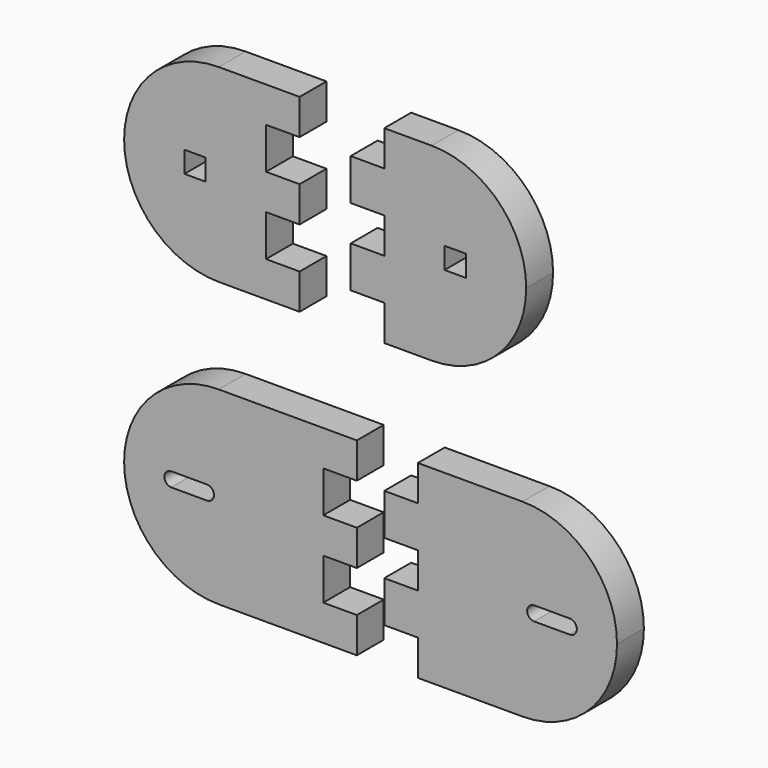
from build123d import *

# Parameters (mm, degrees)
F1_W     = 11.43
F1_H     = 11.43
F1_W_2   = 18.034
F1_H_2   = 19.05
F2_DEPTH = 18.034
F1_H_3   = 22.225


# Not quite as in the source:
# - a variable given as a bare number and used for a length is read in inches; the dataset says mm whatever the document's units were
# - a feature names something its author has since deleted; it is built from what else it names


with BuildPart() as f2:
    # F1 (on Front) → F2 (new body)
    with BuildSketch(Plane.XZ):
        with BuildLine():
            Line((-25.4, 0), (0, 0))
            Line((0, 0), (0, 19.05))
            Line((0, 19.05), (0, 41.275))
            Line((0, 41.275), (0, 60.325))
            Line((0, 60.325), (0, 82.55))
            Line((0, 82.55), (0, 101.6))
            Line((0, 101.6), (-25.4, 101.6))
            ThreePointArc((-25.4, 101.6), (-61.3210244843, 86.7210244843), (-76.2, 50.8))
            ThreePointArc((-76.2, 50.8), (-61.3210244843, 14.8789755157), (-25.4, 0))
        make_face()
        with Locations((-38.1, 50.8)):
            Rectangle(F1_W, F1_H, mode=Mode.SUBTRACT)
        with Locations((9.017, 92.075)):
            Rectangle(F1_W_2, F1_H_2)
        with Locations((9.017, 50.8)):
            Rectangle(F1_W_2, F1_H_2)
        with Locations((9.017, 9.525)):
            Rectangle(F1_W_2, F1_H_2)
    extrude(amount=F2_DEPTH)


with BuildPart() as f2b:
    # F1 (on Front) → F2, piece 2 (new body)
    with BuildSketch(Plane.XZ):
        with Locations((54.483, 30.1625)):
            Rectangle(F1_W_2, F1_H_3)
        with Locations((54.483, 71.4375)):
            Rectangle(F1_W_2, F1_H_3)
        with BuildLine():
            ThreePointArc((139.7, 50.8), (124.8210244843, 86.7210244843), (88.9, 101.6))
            Line((88.9, 101.6), (63.5, 101.6))
            Line((63.5, 101.6), (63.5, 82.55))
            Line((63.5, 82.55), (63.5, 60.325))
            Line((63.5, 60.325), (63.5, 41.275))
            Line((63.5, 41.275), (63.5, 19.05))
            Line((63.5, 19.05), (63.5, 0))
            Line((63.5, 0), (88.9, 0))
            ThreePointArc((88.9, 0), (124.8210244843, 14.8789755157), (139.7, 50.8))
        make_face()
        with Locations((101.6, 50.8)):
            Rectangle(F1_W, F1_H, mode=Mode.SUBTRACT)
    extrude(amount=F2_DEPTH)


with BuildPart() as f2c:
    # F1 (on Front) → F2, piece 3 (new body)
    with BuildSketch(Plane.XZ):
        with Locations((39.751, -101.6)):
            Rectangle(F1_W_2, F1_H_2)
        with BuildLine():
            Line((30.734, -50.8), (-25.4, -50.8))
            ThreePointArc((-25.4, -50.8), (-61.3210244843, -65.6789755157), (-76.2, -101.6))
            ThreePointArc((-76.2, -101.6), (-61.3210244843, -137.5210244843), (-25.4, -152.4))
            Line((-25.4, -152.4), (30.734, -152.4))
            Line((30.734, -152.4), (30.734, -133.35))
            Line((30.734, -133.35), (30.734, -111.125))
            Line((30.734, -111.125), (30.734, -92.075))
            Line((30.734, -92.075), (30.734, -69.85))
            Line((30.734, -69.85), (30.734, -50.8))
        make_face()
        with BuildLine():
            Line((-31.75, -105.41), (-50.8, -105.41))
            ThreePointArc((-50.8, -105.41), (-54.61, -101.6), (-50.8, -97.79))
            Line((-50.8, -97.79), (-31.75, -97.79))
            ThreePointArc((-31.75, -97.79), (-27.94, -101.6), (-31.75, -105.41))
        make_face(mode=Mode.SUBTRACT)
        with Locations((39.751, -142.875)):
            Rectangle(F1_W_2, F1_H_2)
        with Locations((39.751, -60.325)):
            Rectangle(F1_W_2, F1_H_2)
    extrude(amount=F2_DEPTH)


with BuildPart() as f2d:
    # F1 (on Front) → F2, piece 4 (new body)
    with BuildSketch(Plane.XZ):
        with Locations((72.517, -80.9625)):
            Rectangle(F1_W_2, F1_H_3)
        with Locations((72.517, -122.2375)):
            Rectangle(F1_W_2, F1_H_3)
        with BuildLine():
            Line((137.668, -50.8), (81.534, -50.8))
            Line((81.534, -50.8), (81.534, -69.85))
            Line((81.534, -69.85), (81.534, -92.075))
            Line((81.534, -92.075), (81.534, -111.125))
            Line((81.534, -111.125), (81.534, -133.35))
            Line((81.534, -133.35), (81.534, -152.4))
            Line((81.534, -152.4), (137.668, -152.4))
            ThreePointArc((137.668, -152.4), (173.5890244843, -137.5210244843), (188.468, -101.6))
            ThreePointArc((188.468, -101.6), (173.5890244843, -65.6789755157), (137.668, -50.8))
        make_face()
        with BuildLine():
            ThreePointArc((144.018, -105.41), (140.208, -101.6), (144.018, -97.79))
            Line((144.018, -97.79), (163.068, -97.79))
            ThreePointArc((163.068, -97.79), (166.878, -101.6), (163.068, -105.41))
            Line((163.068, -105.41), (144.018, -105.41))
        make_face(mode=Mode.SUBTRACT)
    extrude(amount=F2_DEPTH)


solid = Compound([f2.part, f2b.part, f2c.part, f2d.part])
